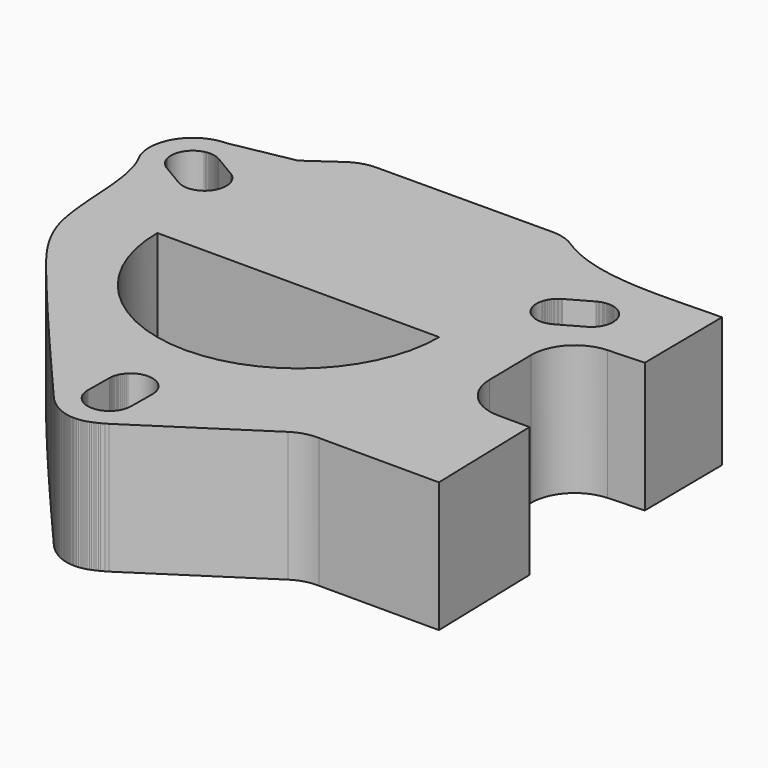
from build123d import *

# Parameters (mm, degrees)
F1_DEPTH = 30
F3_DEPTH = 30
F5_DEPTH = 3


# Not quite as in the source:
# - ends of sketch curves that miss each other by under 0.0002 mm in the source are joined


with BuildPart() as f1:
    # F0 (on Top) → F1 (new body)
    with BuildSketch(Plane.XY):
        with BuildLine():
            Line((-37.064599, 48.313191), (-51.2810601346, 45.6103825108))
            ThreePointArc((-51.2810601346, 45.6103825108), (-58.2599620866, 42.6319725636), (-61.138762, 35.611395))
            Line((-61.138762, 35.611395), (-61.126391, 35.109443))
            Line((-61.126391, 35.109443), (-61.089704, 34.614046))
            Line((-61.089704, 34.614046), (-61.029339, 34.125931))
            Line((-61.029339, 34.125931), (-60.945935, 33.645826))
            Line((-60.945935, 33.645826), (-60.840129, 33.174457))
            Line((-60.840129, 33.174457), (-60.712559, 32.712551))
            Line((-60.712559, 32.712551), (-60.563865, 32.260836))
            Line((-60.563865, 32.260836), (-60.394684, 31.820038))
            Line((-60.394684, 31.820038), (-60.202886, 31.478016))
            Line((-60.202886, 31.478016), (-60.019234, 31.130785))
            Line((-60.019234, 31.130785), (-59.843515, 30.778455))
            Line((-59.843515, 30.778455), (-59.675516, 30.421137))
            Line((-59.675516, 30.421137), (-59.515025, 30.058942))
            Line((-59.515025, 30.058942), (-59.361829, 29.69198))
            Line((-59.361829, 29.69198), (-59.215717, 29.320363))
            Line((-59.215717, 29.320363), (-59.076475, 28.944201))
            Line((-59.076475, 28.944201), (-58.943893, 28.563605))
            Line((-58.943893, 28.563605), (-58.817756, 28.178686))
            Line((-58.817756, 28.178686), (-58.583971, 27.396321))
            Line((-58.583971, 27.396321), (-58.373421, 26.597994))
            Line((-58.373421, 26.597994), (-58.184408, 25.784591))
            Line((-58.184408, 25.784591), (-58.015232, 24.956999))
            Line((-58.015232, 24.956999), (-57.864194, 24.116103))
            Line((-57.864194, 24.116103), (-57.729595, 23.262792))
            Line((-57.729595, 23.262792), (-57.609736, 22.39795))
            Line((-57.609736, 22.39795), (-57.502918, 21.522466))
            Line((-57.502918, 21.522466), (-57.407442, 20.637225))
            Line((-57.407442, 20.637225), (-57.321607, 19.743114))
            Line((-57.321607, 19.743114), (-57.243717, 18.841019))
            Line((-57.243717, 18.841019), (-57.104969, 17.016427))
            Line((-57.104969, 17.016427), (-56.977604, 15.17054))
            Line((-56.977604, 15.17054), (-56.84803, 13.310452))
            Line((-56.84803, 13.310452), (-56.702654, 11.443255))
            Line((-56.702654, 11.443255), (-56.619793, 10.509207))
            Line((-56.619793, 10.509207), (-56.527883, 9.576041))
            Line((-56.527883, 9.576041), (-56.425226, 8.644644))
            Line((-56.425226, 8.644644), (-56.310123, 7.715904))
            Line((-56.310123, 7.715904), (-56.180874, 6.790705))
            Line((-56.180874, 6.790705), (-56.035781, 5.869935))
            Line((-56.035781, 5.869935), (-55.873144, 4.954481))
            Line((-55.873144, 4.954481), (-55.691265, 4.045229))
            Line((-55.691265, 4.045229), (-55.553458, 3.436864))
            Line((-55.553458, 3.436864), (-55.399542, 2.833928))
            Line((-55.399542, 2.833928), (-55.230064, 2.236351))
            Line((-55.230064, 2.236351), (-55.04557, 1.644065))
            Line((-55.04557, 1.644065), (-54.846607, 1.057004))
            Line((-54.846607, 1.057004), (-54.633721, 0.475098))
            Line((-54.633721, 0.475098), (-54.407458, -0.101721))
            Line((-54.407458, -0.101721), (-54.168365, -0.673521))
            Line((-54.168365, -0.673521), (-53.916987, -1.240369))
            Line((-53.916987, -1.240369), (-53.653873, -1.802334))
            Line((-53.653873, -1.802334), (-53.379566, -2.359484))
            Line((-53.379566, -2.359484), (-53.094615, -2.911888))
            Line((-53.094615, -2.911888), (-52.799565, -3.459613))
            Line((-52.799565, -3.459613), (-52.494963, -4.002727))
            Line((-52.494963, -4.002727), (-52.181355, -4.541299))
            Line((-52.181355, -4.541299), (-51.859287, -5.075396))
            Line((-51.859287, -5.075396), (-51.529307, -5.605087))
            Line((-51.529307, -5.605087), (-51.191959, -6.13044))
            Line((-51.191959, -6.13044), (-50.847791, -6.651523))
            Line((-50.847791, -6.651523), (-50.497348, -7.168404))
            Line((-50.497348, -7.168404), (-49.779827, -8.189832))
            Line((-49.779827, -8.189832), (-49.043765, -9.19527))
            Line((-49.043765, -9.19527), (-48.293533, -10.185262))
            Line((-48.293533, -10.185262), (-47.533502, -11.160354))
            Line((-47.533502, -11.160354), (-46.768043, -12.12109))
            Line((-46.768043, -12.12109), (-46.001527, -13.068015))
            Line((-46.001527, -13.068015), (-43.947915, -15.580125))
            Line((-43.947915, -15.580125), (-41.875962, -18.096015))
            Line((-41.875962, -18.096015), (-39.789943, -20.611975))
            Line((-39.789943, -20.611975), (-37.694131, -23.124298))
            Line((-37.694131, -23.124298), (-35.592801, -25.629274))
            Line((-35.592801, -25.629274), (-33.490227, -28.123193))
            Line((-33.490227, -28.123193), (-29.298444, -33.063027))
            Line((-29.298444, -33.063027), (-25.152975, -37.914128))
            Line((-25.152975, -37.914128), (-21.088013, -42.646824))
            Line((-21.088013, -42.646824), (-13.336389, -51.638312))
            Line((-13.336389, -51.638312), (-12.934549, -52.028145))
            Line((-12.934549, -52.028145), (-12.524259, -52.401363))
            Line((-12.524259, -52.401363), (-12.105122, -52.756788))
            Line((-12.105122, -52.756788), (-11.676741, -53.093243))
            Line((-11.676741, -53.093243), (-11.238717, -53.409551))
            Line((-11.238717, -53.409551), (-10.790653, -53.704532))
            Line((-10.790653, -53.704532), (-10.332153, -53.977009))
            Line((-10.332153, -53.977009), (-9.862818, -54.225806))
            Line((-9.862818, -54.225806), (-9.382251, -54.449742))
            Line((-9.382251, -54.449742), (-8.890054, -54.647642))
            Line((-8.890054, -54.647642), (-8.639471, -54.73646))
            Line((-8.639471, -54.73646), (-8.385831, -54.818327))
            Line((-8.385831, -54.818327), (-8.129085, -54.893096))
            Line((-8.129085, -54.893096), (-7.869183, -54.96062))
            Line((-7.869183, -54.96062), (-7.606076, -55.020751))
            Line((-7.606076, -55.020751), (-7.339714, -55.073342))
            Line((-7.339714, -55.073342), (-7.070046, -55.118246))
            Line((-7.070046, -55.118246), (-6.797024, -55.155316))
            Line((-6.797024, -55.155316), (-6.520598, -55.184405))
            Line((-6.520598, -55.184405), (-6.240719, -55.205364))
            Line((-6.240719, -55.205364), (-5.957335, -55.218048))
            Line((-5.957335, -55.218048), (-5.670399, -55.222309))
            Line((-5.670399, -55.222309), (-5.233905, -55.209095))
            Line((-5.233905, -55.209095), (-4.802755, -55.170733))
            Line((-4.802755, -55.170733), (-4.377204, -55.109141))
            Line((-4.377204, -55.109141), (-3.957511, -55.026238))
            Line((-3.957511, -55.026238), (-3.543933, -54.923942))
            Line((-3.543933, -54.923942), (-3.136727, -54.804171))
            Line((-3.136727, -54.804171), (-2.736152, -54.668845))
            Line((-2.736152, -54.668845), (-2.342463, -54.519882))
            Line((-2.342463, -54.519882), (-1.95592, -54.359199))
            Line((-1.95592, -54.359199), (-1.576779, -54.188717))
            Line((-1.576779, -54.188717), (-1.205299, -54.010353))
            Line((-1.205299, -54.010353), (-0.841735, -53.826025))
            Line((-0.841735, -53.826025), (-0.13939, -53.447155))
            Line((-0.13939, -53.447155), (0.528195, -53.067454))
            Line((0.528195, -53.067454), (27.64216, -35.379145))
            ThreePointArc((27.64216, -35.379145), (30.4271484557, -34.1232689781), (33.4613450137, -33.766846623))
            Line((33.4613450137, -33.766846623), (61.138761, -33.794458))
            Line((61.138761, -33.794458), (60.413353, -6.768427))
            Line((60.413353, -6.768427), (53.311347, -6.768427))
            ThreePointArc((53.311347, -6.768427), (46.2641655311, -3.9068031429), (43.2684581259, 3.0844340019))
            Line((43.2684581259, 3.0844340019), (43.088603, 15.314623))
            ThreePointArc((43.088603, 15.314623), (45.8166154823, 22.2896486263), (52.6233669924, 25.4139361624))
            Line((52.6233669924, 25.4139361624), (60.943439, 25.800928))
            Line((60.943439, 25.800928), (60.723573, 48.291206))
            Line((60.723573, 48.291206), (59.571848, 48.285691))
            Line((59.571848, 48.285691), (58.400739, 48.270528))
            Line((58.400739, 48.270528), (56.00627, 48.219556))
            Line((56.00627, 48.219556), (53.551976, 48.154887))
            Line((53.551976, 48.154887), (51.049669, 48.093116))
            Line((51.049669, 48.093116), (48.511156, 48.05084))
            Line((48.511156, 48.05084), (47.232014, 48.042198))
            Line((47.232014, 48.042198), (45.948249, 48.044652))
            Line((45.948249, 48.044652), (44.661337, 48.060279))
            Line((44.661337, 48.060279), (43.372756, 48.09115))
            Line((43.372756, 48.09115), (42.083981, 48.139343))
            Line((42.083981, 48.139343), (40.796488, 48.20693))
            Line((40.796488, 48.20693), (39.511753, 48.295986))
            Line((39.511753, 48.295986), (38.231254, 48.408585))
            Line((38.231254, 48.408585), (36.956466, 48.546803))
            Line((36.956466, 48.546803), (35.688864, 48.712714))
            Line((35.688864, 48.712714), (35.05822, 48.806702))
            Line((35.05822, 48.806702), (34.429927, 48.908391))
            Line((34.429927, 48.908391), (33.804168, 49.018041))
            Line((33.804168, 49.018041), (33.181129, 49.13591))
            Line((33.181129, 49.13591), (32.560994, 49.262258))
            Line((32.560994, 49.262258), (31.943947, 49.397345))
            Line((31.943947, 49.397345), (31.330173, 49.541429))
            Line((31.330173, 49.541429), (30.719857, 49.69477))
            Line((30.719857, 49.69477), (30.113183, 49.857627))
            Line((30.113183, 49.857627), (29.510336, 50.03026))
            Line((29.510336, 50.03026), (28.911499, 50.212928))
            Line((28.911499, 50.212928), (28.316859, 50.405889))
            Line((28.316859, 50.405889), (27.726598, 50.609405))
            Line((27.726598, 50.609405), (27.140903, 50.823733))
            Line((27.140903, 50.823733), (26.559956, 51.049133))
            Line((26.559956, 51.049133), (25.983944, 51.285864))
            Line((25.983944, 51.285864), (25.41305, 51.534186))
            Line((25.41305, 51.534186), (24.847458, 51.794358))
            Line((24.847458, 51.794358), (24.287354, 52.06664))
            Line((24.287354, 52.06664), (23.732922, 52.35129))
            Line((23.732922, 52.35129), (23.184346, 52.648567))
            Line((23.184346, 52.648567), (22.641812, 52.958732))
            Line((22.641812, 52.958732), (22.105502, 53.282044))
            Line((22.105502, 53.282044), (21.575603, 53.618762))
            ThreePointArc((21.575603, 53.618762), (18.9537369154, 54.8195548193), (16.0982230022, 55.2222025272))
            Line((16.0982230022, 55.2222025272), (-24.401708, 55.03554))
            ThreePointArc((-24.401708, 55.03554), (-27.3634481093, 54.5594371392), (-30.0507269762, 53.2263539661))
            Line((-30.0507269762, 53.2263539661), (-37.064599, 48.313191))
        make_face()
        with BuildLine():
            Line((-10.670084, -45.166241), (-10.602282, -39.12079))
            Line((-10.602282, -39.12079), (-10.59387, -38.881015))
            Line((-10.59387, -38.881015), (-10.574023, -38.641813))
            Line((-10.574023, -38.641813), (-10.542746, -38.403629))
            Line((-10.542746, -38.403629), (-10.500043, -38.166906))
            Line((-10.500043, -38.166906), (-10.44592, -37.932089))
            Line((-10.44592, -37.932089), (-10.380382, -37.699621))
            Line((-10.380382, -37.699621), (-10.303434, -37.469948))
            Line((-10.303434, -37.469948), (-10.21508, -37.243513))
            Line((-10.21508, -37.243513), (-10.115326, -37.020761))
            Line((-10.115326, -37.020761), (-10.004177, -36.802136))
            Line((-10.004177, -36.802136), (-9.881637, -36.588081))
            Line((-9.881637, -36.588081), (-9.747713, -36.379042))
            Line((-9.747713, -36.379042), (-9.602407, -36.175463))
            Line((-9.602407, -36.175463), (-9.445726, -35.977787))
            Line((-9.445726, -35.977787), (-9.277675, -35.786459))
            Line((-9.277675, -35.786459), (-9.098258, -35.601923))
            ThreePointArc((-9.098258, -35.601923), (-5.5465234312, -34.1771984344), (-2.0276354376, -35.6812224278))
            Line((-2.0276354376, -35.6812224278), (-1.852402, -35.869737))
            Line((-1.852402, -35.869737), (-1.688683, -36.064787))
            Line((-1.688683, -36.064787), (-1.536475, -36.265928))
            Line((-1.536475, -36.265928), (-1.395771, -36.472717))
            Line((-1.395771, -36.472717), (-1.266568, -36.684708))
            Line((-1.266568, -36.684708), (-1.14886, -36.901458))
            Line((-1.14886, -36.901458), (-1.042641, -37.122522))
            Line((-1.042641, -37.122522), (-0.947908, -37.347456))
            Line((-0.947908, -37.347456), (-0.864655, -37.575816))
            Line((-0.864655, -37.575816), (-0.792878, -37.807158))
            Line((-0.792878, -37.807158), (-0.73257, -38.041037))
            Line((-0.73257, -38.041037), (-0.683728, -38.27701))
            Line((-0.683728, -38.27701), (-0.646346, -38.514631))
            Line((-0.646346, -38.514631), (-0.620419, -38.753457))
            Line((-0.620419, -38.753457), (-0.605942, -38.993044))
            Line((-0.605942, -38.993044), (-0.602911, -39.232946))
            Line((-0.602911, -39.232946), (-0.670713, -45.278386))
            Line((-0.670713, -45.278386), (-0.679123, -45.518161))
            Line((-0.679123, -45.518161), (-0.698969, -45.757362))
            Line((-0.698969, -45.757362), (-0.730246, -45.995546))
            Line((-0.730246, -45.995546), (-0.772947, -46.23227))
            Line((-0.772947, -46.23227), (-0.827069, -46.467088))
            Line((-0.827069, -46.467088), (-0.892607, -46.699556))
            Line((-0.892607, -46.699556), (-0.969555, -46.92923))
            Line((-0.969555, -46.92923), (-1.057909, -47.155666))
            Line((-1.057909, -47.155666), (-1.157663, -47.37842))
            Line((-1.157663, -47.37842), (-1.268812, -47.597047))
            Line((-1.268812, -47.597047), (-1.391352, -47.811103))
            Line((-1.391352, -47.811103), (-1.525278, -48.020144))
            Line((-1.525278, -48.020144), (-1.670584, -48.223725))
            Line((-1.670584, -48.223725), (-1.827266, -48.421403))
            Line((-1.827266, -48.421403), (-1.995319, -48.612733))
            Line((-1.995319, -48.612733), (-2.174737, -48.79727))
            ThreePointArc((-2.174737, -48.79727), (-5.7264718618, -50.2219945735), (-9.2453600737, -48.717971072))
            Line((-9.2453600737, -48.717971072), (-9.420594, -48.529456))
            Line((-9.420594, -48.529456), (-9.584313, -48.334405))
            Line((-9.584313, -48.334405), (-9.736522, -48.133263))
            Line((-9.736522, -48.133263), (-9.877226, -47.926474))
            Line((-9.877226, -47.926474), (-10.006429, -47.714482))
            Line((-10.006429, -47.714482), (-10.124138, -47.497732))
            Line((-10.124138, -47.497732), (-10.230356, -47.276667))
            Line((-10.230356, -47.276667), (-10.325089, -47.051732))
            Line((-10.325089, -47.051732), (-10.408342, -46.823372))
            Line((-10.408342, -46.823372), (-10.48012, -46.592029))
            Line((-10.48012, -46.592029), (-10.540427, -46.35815))
            Line((-10.540427, -46.35815), (-10.589269, -46.122177))
            Line((-10.589269, -46.122177), (-10.626651, -45.884556))
            Line((-10.626651, -45.884556), (-10.652577, -45.64573))
            Line((-10.652577, -45.64573), (-10.667053, -45.406143))
            Line((-10.667053, -45.406143), (-10.670084, -45.166241))
        make_face(mode=Mode.SUBTRACT)
        with BuildLine():
            ThreePointArc((-39.181587, 10.445087), (-29.6625573886, 33.4260573886), (-6.681587, 42.945087))
            ThreePointArc((-6.681587, 42.945087), (16.2993833886, 33.4260573886), (25.818413, 10.445087))
            ThreePointArc((25.818413, 10.445087), (16.2993833886, -12.5358833886), (-6.681587, -22.054913))
            ThreePointArc((-6.681587, -22.054913), (-29.6625573886, -12.5358833886), (-39.181587, 10.445087))
        make_face(mode=Mode.SUBTRACT)
        with BuildLine():
            Line((-48.590362, 39.913216), (-43.388749, 36.831772))
            Line((-43.388749, 36.831772), (-43.185304, 36.7046))
            Line((-43.185304, 36.7046), (-42.988073, 36.567811))
            Line((-42.988073, 36.567811), (-42.797438, 36.421631))
            Line((-42.797438, 36.421631), (-42.613781, 36.266288))
            Line((-42.613781, 36.266288), (-42.437485, 36.102008))
            Line((-42.437485, 36.102008), (-42.268931, 35.929017))
            Line((-42.268931, 35.929017), (-42.108503, 35.747541))
            Line((-42.108503, 35.747541), (-41.956581, 35.557807))
            Line((-41.956581, 35.557807), (-41.813549, 35.360041))
            Line((-41.813549, 35.360041), (-41.679789, 35.154471))
            Line((-41.679789, 35.154471), (-41.555682, 34.941321))
            Line((-41.555682, 34.941321), (-41.441611, 34.720819))
            Line((-41.441611, 34.720819), (-41.337959, 34.493191))
            Line((-41.337959, 34.493191), (-41.245107, 34.258664))
            Line((-41.245107, 34.258664), (-41.163437, 34.017463))
            Line((-41.163437, 34.017463), (-41.093333, 33.769816))
            ThreePointArc((-41.093333, 33.769816), (-41.6353527547, 29.9815606205), (-44.6973199274, 27.6861257164))
            Line((-44.6973199274, 27.6861257164), (-44.948195, 27.628627))
            Line((-44.948195, 27.628627), (-45.198973, 27.584367))
            Line((-45.198973, 27.584367), (-45.44927, 27.553121))
            Line((-45.44927, 27.553121), (-45.698706, 27.534663))
            Line((-45.698706, 27.534663), (-45.946897, 27.528765))
            Line((-45.946897, 27.528765), (-46.193462, 27.535202))
            Line((-46.193462, 27.535202), (-46.438019, 27.553746))
            Line((-46.438019, 27.553746), (-46.680184, 27.584172))
            Line((-46.680184, 27.584172), (-46.919576, 27.626253))
            Line((-46.919576, 27.626253), (-47.155813, 27.679763))
            Line((-47.155813, 27.679763), (-47.388512, 27.744474))
            Line((-47.388512, 27.744474), (-47.617291, 27.820162))
            Line((-47.617291, 27.820162), (-47.841769, 27.906599))
            Line((-47.841769, 27.906599), (-48.061561, 28.003558))
            Line((-48.061561, 28.003558), (-48.276288, 28.110815))
            Line((-48.276288, 28.110815), (-48.485565, 28.228141))
            Line((-48.485565, 28.228141), (-53.687169, 31.309579))
            Line((-53.687169, 31.309579), (-53.890614, 31.43675))
            Line((-53.890614, 31.43675), (-54.087846, 31.573537))
            Line((-54.087846, 31.573537), (-54.278481, 31.719716))
            Line((-54.278481, 31.719716), (-54.462139, 31.875058))
            Line((-54.462139, 31.875058), (-54.638436, 32.039338))
            Line((-54.638436, 32.039338), (-54.806991, 32.21233))
            Line((-54.806991, 32.21233), (-54.96742, 32.393806))
            Line((-54.96742, 32.393806), (-55.119343, 32.58354))
            Line((-55.119343, 32.58354), (-55.262376, 32.781306))
            Line((-55.262376, 32.781306), (-55.396138, 32.986878))
            Line((-55.396138, 32.986878), (-55.520246, 33.200029))
            Line((-55.520246, 33.200029), (-55.634318, 33.420533))
            Line((-55.634318, 33.420533), (-55.737971, 33.648162))
            Line((-55.737971, 33.648162), (-55.830824, 33.882692))
            Line((-55.830824, 33.882692), (-55.912495, 34.123894))
            Line((-55.912495, 34.123894), (-55.9826, 34.371544))
            ThreePointArc((-55.9826, 34.371544), (-55.4405799984, 38.1597987962), (-52.3786130726, 40.4552332836))
            Line((-52.3786130726, 40.4552332836), (-52.127737, 40.512733))
            Line((-52.127737, 40.512733), (-51.876958, 40.556992))
            Line((-51.876958, 40.556992), (-51.62666, 40.588238))
            Line((-51.62666, 40.588238), (-51.377224, 40.606697))
            Line((-51.377224, 40.606697), (-51.129031, 40.612594))
            Line((-51.129031, 40.612594), (-50.882466, 40.606158))
            Line((-50.882466, 40.606158), (-50.637909, 40.587613))
            Line((-50.637909, 40.587613), (-50.395743, 40.557187))
            Line((-50.395743, 40.557187), (-50.156351, 40.515106))
            Line((-50.156351, 40.515106), (-49.920114, 40.461596))
            Line((-49.920114, 40.461596), (-49.687414, 40.396884))
            Line((-49.687414, 40.396884), (-49.458635, 40.321196))
            Line((-49.458635, 40.321196), (-49.234158, 40.234759))
            Line((-49.234158, 40.234759), (-49.014365, 40.137799))
            Line((-49.014365, 40.137799), (-48.799639, 40.030542))
            Line((-48.799639, 40.030542), (-48.590362, 39.913216))
        make_face(mode=Mode.SUBTRACT)
        with BuildLine():
            Line((44.050747, 30.213412), (38.781332, 27.249405))
            Line((38.781332, 27.249405), (38.569475, 27.136802))
            Line((38.569475, 27.136802), (38.352397, 27.034389))
            Line((38.352397, 27.034389), (38.130484, 26.942384))
            Line((38.130484, 26.942384), (37.904125, 26.861004))
            Line((37.904125, 26.861004), (37.673706, 26.790467))
            Line((37.673706, 26.790467), (37.439614, 26.730991))
            Line((37.439614, 26.730991), (37.202237, 26.682794))
            Line((37.202237, 26.682794), (36.961962, 26.646093))
            Line((36.961962, 26.646093), (36.719176, 26.621106))
            Line((36.719176, 26.621106), (36.474266, 26.608052))
            Line((36.474266, 26.608052), (36.22762, 26.607147))
            Line((36.22762, 26.607147), (35.979624, 26.61861))
            Line((35.979624, 26.61861), (35.730667, 26.642658))
            Line((35.730667, 26.642658), (35.481134, 26.67951))
            Line((35.481134, 26.67951), (35.231413, 26.729382))
            Line((35.231413, 26.729382), (34.981892, 26.792494))
            ThreePointArc((34.981892, 26.792494), (31.9721773874, 29.1560245611), (31.5152565247, 32.9554828531))
            Line((31.5152565247, 32.9554828531), (31.590898, 33.201497))
            Line((31.590898, 33.201497), (31.677957, 33.440806))
            Line((31.677957, 33.440806), (31.776046, 33.673193))
            Line((31.776046, 33.673193), (31.884778, 33.89844))
            Line((31.884778, 33.89844), (32.003766, 34.116329))
            Line((32.003766, 34.116329), (32.132623, 34.326642))
            Line((32.132623, 34.326642), (32.270961, 34.529162))
            Line((32.270961, 34.529162), (32.418393, 34.723671))
            Line((32.418393, 34.723671), (32.574533, 34.90995))
            Line((32.574533, 34.90995), (32.738992, 35.087782))
            Line((32.738992, 35.087782), (32.911383, 35.256949))
            Line((32.911383, 35.256949), (33.09132, 35.417234))
            Line((33.09132, 35.417234), (33.278415, 35.568419))
            Line((33.278415, 35.568419), (33.472281, 35.710285))
            Line((33.472281, 35.710285), (33.672531, 35.842616))
            Line((33.672531, 35.842616), (33.878777, 35.965192))
            Line((33.878777, 35.965192), (39.148183, 38.929194))
            Line((39.148183, 38.929194), (39.360038, 39.041797))
            Line((39.360038, 39.041797), (39.577116, 39.144211))
            Line((39.577116, 39.144211), (39.799028, 39.236217))
            Line((39.799028, 39.236217), (40.025387, 39.317598))
            Line((40.025387, 39.317598), (40.255806, 39.388136))
            Line((40.255806, 39.388136), (40.489899, 39.447613))
            Line((40.489899, 39.447613), (40.727276, 39.495811))
            Line((40.727276, 39.495811), (40.967552, 39.532513))
            Line((40.967552, 39.532513), (41.21034, 39.5575))
            Line((41.21034, 39.5575), (41.455251, 39.570555))
            Line((41.455251, 39.570555), (41.701899, 39.57146))
            Line((41.701899, 39.57146), (41.949897, 39.559998))
            Line((41.949897, 39.559998), (42.198857, 39.535949))
            Line((42.198857, 39.535949), (42.448391, 39.499098))
            Line((42.448391, 39.499098), (42.698114, 39.449225))
            Line((42.698114, 39.449225), (42.947637, 39.386113))
            ThreePointArc((42.947637, 39.386113), (45.9573521405, 37.0225822782), (46.4142736623, 33.2231238146))
            Line((46.4142736623, 33.2231238146), (46.338632, 32.977109))
            Line((46.338632, 32.977109), (46.251572, 32.737799))
            Line((46.251572, 32.737799), (46.153483, 32.505411))
            Line((46.153483, 32.505411), (46.04475, 32.280164))
            Line((46.04475, 32.280164), (45.925762, 32.062274))
            Line((45.925762, 32.062274), (45.796904, 31.851961))
            Line((45.796904, 31.851961), (45.658566, 31.64944))
            Line((45.658566, 31.64944), (45.511133, 31.454932))
            Line((45.511133, 31.454932), (45.354993, 31.268652))
            Line((45.354993, 31.268652), (45.190534, 31.09082))
            Line((45.190534, 31.09082), (45.018142, 30.921653))
            Line((45.018142, 30.921653), (44.838205, 30.761368))
            Line((44.838205, 30.761368), (44.65111, 30.610184))
            Line((44.65111, 30.610184), (44.457243, 30.468318))
            Line((44.457243, 30.468318), (44.256994, 30.335988))
            Line((44.256994, 30.335988), (44.050747, 30.213412))
        make_face(mode=Mode.SUBTRACT)
    extrude(amount=F1_DEPTH)

    # F2 (on face) → F3 (join)
    with BuildSketch(Plane.XY):
        with BuildLine():
            ThreePointArc((-39.1141668096, 12.5373983756), (-39.1645580744, 11.4970329009), (-39.1815853039, 10.4555869475))
            Line((-39.1815853039, 10.4555869475), (25.8184113039, 10.4555869475))
            ThreePointArc((25.8184113039, 10.4555869475), (25.8013840744, 11.4970329009), (25.7509928096, 12.5373983756))
            Line((25.7509928096, 12.5373983756), (-39.1141668096, 12.5373983756))
        make_face()
    extrude(amount=F3_DEPTH)

    # F4 (on face) → F5 (join)
    with BuildSketch(Plane.XY.offset(30)):
        with BuildLine():
            ThreePointArc((26.8682856113, 11.6367153823), (-6.8773226812, 45.1158562171), (-40.6229309738, 11.6367153823))
            Line((-40.6229309738, 11.6367153823), (26.8682856113, 11.6367153823))
        make_face()
        with BuildLine():
            Line((25.7509928096, 12.5373983756), (-39.1141668096, 12.5373983756))
            ThreePointArc((-39.1141668096, 12.5373983756), (-6.681587, 42.945087), (25.7509928096, 12.5373983756))
        make_face(mode=Mode.SUBTRACT)
        with BuildLine():
            ThreePointArc((25.7509928096, 12.5373983756), (-6.681587, 42.945087), (-39.1141668096, 12.5373983756))
            Line((-39.1141668096, 12.5373983756), (25.7509928096, 12.5373983756))
        make_face()
    extrude(amount=-F5_DEPTH)


solid = f1.part
